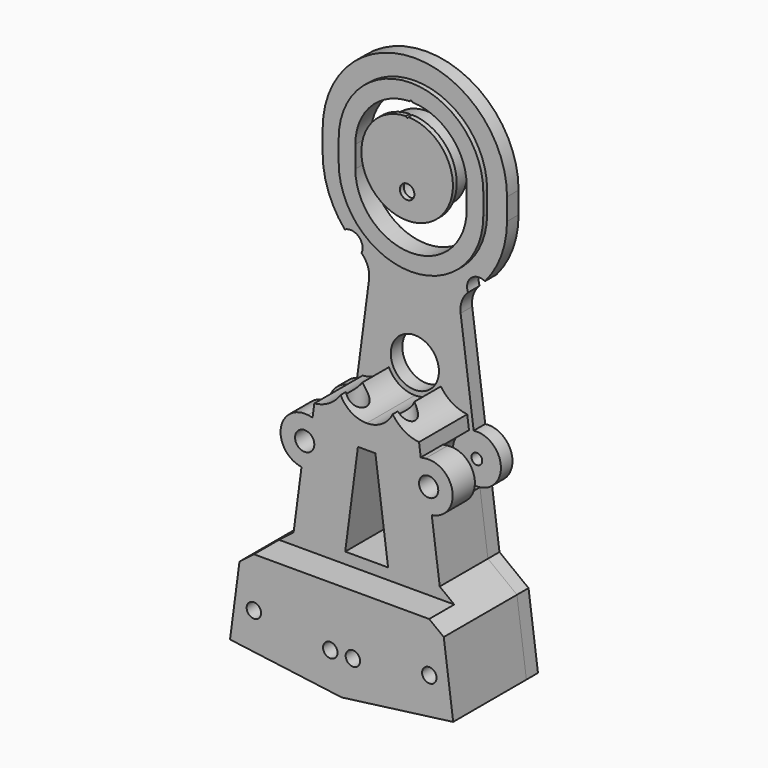
from build123d import *
from build123d import SkipClean  # not in build123d's __all__

# Parameters (mm, degrees)
F1_R        = 1.125
F2_DEPTH    = 3
F5_DEPTH    = 3
F6_T1_DEPTH = 3
F7_R        = 1.5
F7_R_2      = 2
F8_DEPTH    = 19
F9_R        = 2
F10_DEPTH   = 6.5
F12_DEPTH   = 6.75
F13_R       = 8
F14_DEPTH   = 12.7
F15_R       = 4
F16_DEPTH   = 3
F17_R       = 2.25
F18_DEPTH   = 95.4762425203
F20_R       = 8.5
F20_R_2     = 2.75
F21_DEPTH   = 4
F22_R       = 1.5
F23_DEPTH   = 1
F25_DEPTH   = 3
F27_DEPTH   = 1


# Not quite as in the source:
# - a fillet or chamfer that OpenCascade refuses, or shapes differently, is made with other operations: its cross-section is extruded or revolved along the edge and cut away or added


with BuildPart() as f2:
    # F1 (on Front) → F2 (new body)
    with BuildSketch(Plane.XZ):
        with BuildLine():
            Line((0, -36.125), (0, -53.4573349107))
            Line((0, -53.4573349107), (23.1527977927, -50.4092112552))
            Line((23.1527977927, -50.4092112552), (21.1949049094, -35.5375383346))
            Line((21.1949049094, -35.5375383346), (15.1643104963, -30.9101004879))
            Line((15.1643104963, -30.9101004879), (13.5164173195, -18.3931091131))
            ThreePointArc((13.5164173195, -18.3931091131), (17.8210106653, -12.7832538451), (12.2111553973, -8.4786604993))
            Line((12.2111553973, -8.4786604993), (9.097402976, 15.1726372606))
            Line((9.097402976, 15.1726372606), (0, 15.1726372606))
            Line((0, 15.1726372606), (0, 5))
            ThreePointArc((0, 5), (5, 0), (0, -5))
            Line((0, -5), (0, -10.9101004879))
            Line((0, -10.9101004879), (1.8145778384, -10.9101004879))
            Line((1.8145778384, -10.9101004879), (4.4476277901, -30.9101004879))
            Line((4.4476277901, -30.9101004879), (0, -30.9101004879))
            Line((0, -30.9101004879), (0, -33.875))
            ThreePointArc((0, -33.875), (1.125, -35), (0, -36.125))
        make_face()
        with Locations((2.3449541235, -45.5838986393)):
            Circle(F1_R, mode=Mode.SUBTRACT)
        with Locations((18.2080719055, -43.4954795638)):
            Circle(F1_R, mode=Mode.SUBTRACT)
        with Locations((12.8637863584, -13.4358848062)):
            Circle(F1_R, mode=Mode.SUBTRACT)
    extrude(amount=F2_DEPTH)

    # F3: F2 across face


with BuildPart() as f2_1:
    add(f2.part, clean=False)
    with SkipClean():  # cleaning this boolean's faces spoils the solid; the shape is the same uncleaned
        add(f2.part.mirror(Plane(origin=(0, -1.5, 10.0863186303), x_dir=(0, -1, 0), z_dir=(-1, 0, 0))), clean=False)

    # F4 (on Front) → F5 (join)
    with BuildSketch(Plane.XZ):
        with BuildLine():
            Line((-9.097402976, 15.1726372606), (9.097402976, 15.1726372606))
            ThreePointArc((9.097402976, 15.1726372606), (10.0927673962, 15.7501100324), (11.0516074637, 16.3863889462))
            ThreePointArc((11.0516074637, 16.3863889462), (11.6564981463, 19.2340907905), (14.5473139303, 19.5783038564))
            ThreePointArc((14.5473139303, 19.5783038564), (17.9471454109, 25.3801171256), (19.1291107392, 32))
            Line((19.1291107392, 32), (19.1291107392, 36.5))
            ThreePointArc((19.1291107392, 36.5), (0, 55.6291107392), (-19.1291107392, 36.5))
            Line((-19.1291107392, 36.5), (-19.1291107392, 32))
            ThreePointArc((-19.1291107392, 32), (-17.9471454109, 25.3801171256), (-14.5473139303, 19.5783038564))
            ThreePointArc((-14.5473139303, 19.5783038564), (-11.6564981463, 19.2340907905), (-11.0516074637, 16.3863889462))
            ThreePointArc((-11.0516074637, 16.3863889462), (-10.0927673962, 15.7501100324), (-9.097402976, 15.1726372606))
        make_face()
        with BuildLine():
            ThreePointArc((-14, 36.5), (0, 50.5), (14, 36.5))
            Line((14, 36.5), (14, 32))
            ThreePointArc((14, 32), (0, 18), (-14, 32))
            Line((-14, 32), (-14, 36.5))
        make_face(mode=Mode.SUBTRACT)
    extrude(amount=F5_DEPTH)

    # F6: fillet of radius 5 on 2 edges, made by hand

    # F6_s2 → F6_t1 (join)
    with BuildSketch(Plane.XZ):
        with BuildLine():
            ThreePointArc((-9.5048895535, 12.0774694136), (-9.7561149052, 14.4193528228), (-11.0516074637, 16.3863889462))
            ThreePointArc((-11.0516074637, 16.3863889462), (-10.0927673962, 15.7501100324), (-9.097402976, 15.1726372606))
            Line((-9.097402976, 15.1726372606), (-9.5048895535, 12.0774694136))
        make_face()
        with BuildLine():
            ThreePointArc((11.0516074637, 16.3863889462), (9.7561149052, 14.4193528228), (9.5048895535, 12.0774694136))
            Line((9.5048895535, 12.0774694136), (9.097402976, 15.1726372606))
            ThreePointArc((9.097402976, 15.1726372606), (10.0927673962, 15.7501100324), (11.0516074637, 16.3863889462))
        make_face()
    extrude(amount=F6_T1_DEPTH)


with BuildPart() as f8:
    # F7 (on face) → F8 (new body)
    with BuildSketch(Plane.XZ.offset(3)):
        with BuildLine():
            Line((0, -30.9101004879), (0, -53.4573349107))
            Line((0, -53.4573349107), (23.1527977927, -50.4092112552))
            Line((23.1527977927, -50.4092112552), (21.1949049094, -35.5375383346))
            Line((21.1949049094, -35.5375383346), (15.1643104963, -30.9101004879))
            Line((15.1643104963, -30.9101004879), (13.5164173195, -18.3931091131))
            ThreePointArc((13.5164173195, -18.3931091131), (17.8210106653, -12.7832538451), (12.2111553973, -8.4786604993))
            Line((12.2111553973, -8.4786604993), (11.2197105359, -8.6091866915))
            Line((11.2197105359, -8.6091866915), (10.8663730105, -5.9253217294))
            ThreePointArc((10.8663730105, -5.9253217294), (7.7631898412, -4.8808921437), (5.4006866643, -2.6139211071))
            ThreePointArc((5.4006866643, -2.6139211071), (3.1871988766, -5.0834794503), (0, -6))
            Line((0, -6), (0, -10.9101004879))
            Line((0, -10.9101004879), (1.8145778384, -10.9101004879))
            Line((1.8145778384, -10.9101004879), (4.4476277901, -30.9101004879))
            Line((4.4476277901, -30.9101004879), (0, -30.9101004879))
        make_face()
        with Locations((2.3449541235, -45.5838986393)):
            Circle(F7_R, mode=Mode.SUBTRACT)
        with Locations((18.2080719055, -43.4954795638)):
            Circle(F7_R, mode=Mode.SUBTRACT)
        with Locations((12.8637863584, -13.4358848062)):
            Circle(F7_R_2, mode=Mode.SUBTRACT)
    extrude(amount=F8_DEPTH)

    # F9 (on face) → F10 (cut)
    with BuildSketch(Plane.XZ.offset(22)):
        with BuildLine():
            Line((0, -30.9101004879), (0, -33.0778472117))
            Line((0, -33.0778472117), (0, -33.2238194112))
            Line((0, -33.2238194112), (18.1796077028, -33.2238194112))
            Line((18.1796077028, -33.2238194112), (15.1643104963, -30.9101004879))
            Line((15.1643104963, -30.9101004879), (13.5164173195, -18.3931091131))
            ThreePointArc((13.5164173195, -18.3931091131), (17.8210106653, -12.7832538451), (12.2111553973, -8.4786604993))
            Line((12.2111553973, -8.4786604993), (11.2197105359, -8.6091866915))
            Line((11.2197105359, -8.6091866915), (10.8663730105, -5.9253217294))
            ThreePointArc((10.8663730105, -5.9253217294), (9.0225328201, -5.4912132292), (7.3462658428, -4.6089854478))
            ThreePointArc((7.3462658428, -4.6089854478), (6.2800026975, -3.7026083348), (5.4006866643, -2.6139211071))
            ThreePointArc((5.4006866643, -2.6139211071), (4.4679552503, -4.00466926), (3.1871988766, -5.0834794503))
            ThreePointArc((3.1871988766, -5.0834794503), (2.7009322, -5.3577014895), (2.1912834778, -5.5855417571))
            ThreePointArc((2.1912834778, -5.5855417571), (1.1150671409, -5.8954749827), (0, -6))
            Line((0, -6), (0, -10.9101004879))
            Line((0, -10.9101004879), (1.8145778384, -10.9101004879))
            Line((1.8145778384, -10.9101004879), (4.4476277901, -30.9101004879))
            Line((4.4476277901, -30.9101004879), (0, -30.9101004879))
        make_face()
        with Locations((12.8637863584, -13.4358848062)):
            Circle(F9_R, mode=Mode.SUBTRACT)
    extrude(amount=-F10_DEPTH, mode=Mode.SUBTRACT)

    # F11 (on face) → F12 (cut)
    with BuildSketch(Plane.XZ.offset(3)):
        with BuildLine():
            ThreePointArc((11.232896359, -8.7093429615), (9.9615846078, -17.5073986522), (17.8637863584, -13.4358848062))
            ThreePointArc((17.8637863584, -13.4358848062), (16.1605154339, -9.6766857688), (12.2111553973, -8.4786604993))
            ThreePointArc((12.2111553973, -8.4786604993), (11.7162147511, -8.5693583852), (11.232896359, -8.7093429615))
        make_face()
        with BuildLine():
            ThreePointArc((11.232896359, -8.7093429615), (11.7162147511, -8.5693583852), (12.2111553973, -8.4786604993))
            Line((12.2111553973, -8.4786604993), (11.2197105359, -8.6091866915))
            Line((11.2197105359, -8.6091866915), (11.232896359, -8.7093429615))
        make_face()
    extrude(amount=F12_DEPTH, mode=Mode.SUBTRACT)

    # F13 (on face) → F14 (cut)
    with BuildSketch(Plane(origin=(6.9178881876, 0, -52.5465776528), x_dir=(0.9914448614, 0, 0.1305261922), z_dir=(0.1305261922, 0, -0.9914448614))):
        with Locations((4.3724176279, 12)):
            Circle(F13_R)
    extrude(amount=-F14_DEPTH, mode=Mode.SUBTRACT)

    # F15 (on face) → F16 (cut)
    with BuildSketch(Plane(origin=(5.2602055465, 0, -39.9552279134), x_dir=(0.9914448614, 0, 0.1305261922), z_dir=(0.1305261922, 0, -0.9914448614))):
        with Locations((4.3724176279, 12)):
            Circle(F15_R)
    extrude(amount=-F16_DEPTH, mode=Mode.SUBTRACT)

    # F17 (on face) → F18 (cut, through all)
    with BuildSketch(Plane(origin=(4.8686269698, 0, -36.9808933292), x_dir=(0.9914448614, 0, 0.1305261922), z_dir=(0.1305261922, 0, -0.9914448614))):
        with Locations((4.3724176279, 12)):
            Circle(F17_R)
    extrude(amount=-F18_DEPTH, mode=Mode.SUBTRACT)

    # F19: F8 across face


with BuildPart() as f8_1:
    add(f8.part, clean=False)
    add(f8.part.mirror(Plane(origin=(0, -9.25, -8.4550502439), x_dir=(0, -1, 0), z_dir=(-1, 0, 0))), clean=False)


with BuildPart() as f21:
    # F20 (on Front) → F21 (new body)
    with BuildSketch(Plane.XZ):
        with Locations((0, 36.25)):
            Circle(F20_R)
        with Locations((0, 32)):
            Circle(F20_R_2, mode=Mode.SUBTRACT)
    extrude(amount=F21_DEPTH)

    # F22 (on face) → F23 (join)
    with BuildSketch(Plane.XZ.offset(4)):
        with BuildLine():
            ThreePointArc((0.2499783578, 45.7467105263), (0, 45.5), (-0.2499783578, 45.7467105263))
            ThreePointArc((-0.2499783578, 45.7467105263), (0, 26.75), (0.2499783578, 45.7467105263))
        make_face()
        with Locations((0, 32)):
            Circle(F22_R, mode=Mode.SUBTRACT)
    extrude(amount=F23_DEPTH)


with BuildPart() as f25:
    # F24 (on Front) → F25 (new body)
    with BuildSketch(Plane.XZ):
        with BuildLine():
            Line((-14, 36.5), (-14, 32))
            ThreePointArc((-14, 32), (0, 18), (14, 32))
            Line((14, 32), (14, 36.5))
            ThreePointArc((14, 36.5), (0, 50.5), (-14, 36.5))
        make_face()
        with BuildLine():
            ThreePointArc((0.2499853587, 48.0472943723), (8.2549933644, 44.5782166691), (11.55, 36.5))
            Line((11.55, 36.5), (11.55, 32))
            ThreePointArc((11.55, 32), (0, 20.45), (-11.55, 32))
            Line((-11.55, 32), (-11.55, 36.5))
            ThreePointArc((-11.55, 36.5), (-8.2549933644, 44.5782166691), (-0.2499853587, 48.0472943723))
            ThreePointArc((-0.2499853587, 48.0472943723), (0, 48.3), (0.2499853587, 48.0472943723))
        make_face(mode=Mode.SUBTRACT)
    extrude(amount=F25_DEPTH)

    # F26 (on face) → F27 (join)
    with BuildSketch(Plane.XZ.offset(3)):
        with BuildLine():
            Line((-15, 36.5), (-15, 32))
            ThreePointArc((-15, 32), (0, 17), (15, 32))
            Line((15, 32), (15, 36.5))
            ThreePointArc((15, 36.5), (0, 51.5), (-15, 36.5))
        make_face()
        with BuildLine():
            ThreePointArc((0.2499853587, 48.0472943723), (8.2549933644, 44.5782166691), (11.55, 36.5))
            Line((11.55, 36.5), (11.55, 32))
            ThreePointArc((11.55, 32), (0, 20.45), (-11.55, 32))
            Line((-11.55, 32), (-11.55, 36.5))
            ThreePointArc((-11.55, 36.5), (-8.2549933644, 44.5782166691), (-0.2499853587, 48.0472943723))
            ThreePointArc((-0.2499853587, 48.0472943723), (0, 48.3), (0.2499853587, 48.0472943723))
        make_face(mode=Mode.SUBTRACT)
    extrude(amount=F27_DEPTH)


solid = Compound([f2_1.part, f8_1.part, f21.part, f25.part])
